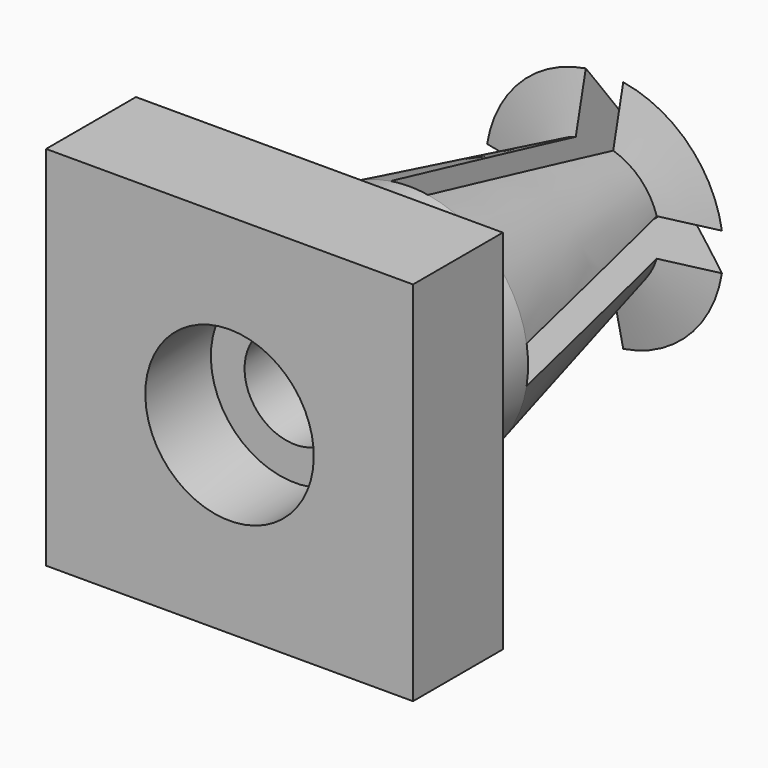
from build123d import *

# Parameters (mm, degrees)
F0_W     = 9.8
F0_H     = 9.8
F0_R     = 2.75
F3_DEPTH = 1.5
F5_START = -4.5
F4_W     = 1
F4_H     = 4.5
F4_H_2   = 1
F4_W_2   = 4.5
F5_DEPTH = 20.5


# Not quite as in the source:
# - a feature names something its author has since deleted; it is built from what else it names


with BuildPart() as f2:
    # F1 (on Right) → F2 (revolve)
    with BuildSketch(Plane.YZ):
        Polygon((4.5, 3.175), (-1.5, 3.175), (-1.5, 2.25), (0.6892941068, 2.25), (0.6892941068, 1.35), (4.0952532458, 1.35), (13.1507472004, 0.5), (11.0196430301, 3.175), (10.6847711314, 1.7358662147), align=None)
    revolve(axis=Axis((0, 11.4737532458, 0), (0, 1, 0)))

    # F0 (on Front) → F3 (join, symmetric)
    with BuildSketch(Plane.XZ):
        Rectangle(F0_W, F0_H)
        Circle(F0_R, mode=Mode.SUBTRACT)
    extrude(amount=F3_DEPTH, both=True)

    # F4 (on Front) → F5 (cut)
    with BuildSketch(Plane.XZ.offset(F5_START)):
        with Locations((0, 2.75)):
            Rectangle(F4_W, F4_H)
        Rectangle(F4_W, F4_H_2)
        with Locations((-2.75, 0)):
            Rectangle(F4_W_2, F4_H_2)
        with Locations((2.75, 0)):
            Rectangle(F4_W_2, F4_H_2)
        with Locations((0, -2.75)):
            Rectangle(F4_W, F4_H)
    extrude(amount=-F5_DEPTH, mode=Mode.SUBTRACT)


solid = f2.part
